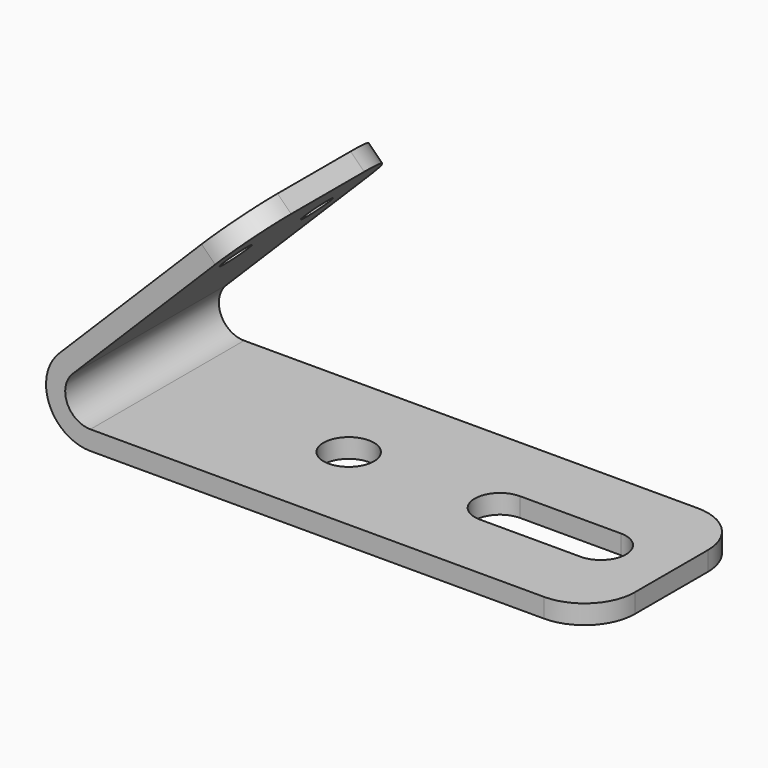
from build123d import *

# Parameters (mm, degrees)
F0_W     = 50
F0_H     = 1.9
F1_DEPTH = 19.05
F3_DEPTH = 1.901
F4_D     = 5
F4_DEPTH = 1.901
F5_R     = 1.5
F6_DEPTH = 15.3122698372
F7_R     = 5


with BuildPart() as f1:
    # F0 (on Front) → F1 (new body)
    with BuildSketch(Plane.XZ):
        with Locations((25, 0.95)):
            Rectangle(F0_W, F0_H)
        with BuildLine():
            ThreePointArc((-3.1112698372, 7.5112698372), (-4.065069943, 2.7161928976), (0, 0))
            Line((0, 0), (0, 1.9))
            ThreePointArc((0, 1.9), (-2.3096988313, 3.4432914191), (-1.767766953, 6.167766953))
            Line((-1.767766953, 6.167766953), (15.9099025767, 23.8454364826))
            Line((15.9099025767, 23.8454364826), (14.5663996924, 25.1889393669))
            Line((14.5663996924, 25.1889393669), (-3.1112698372, 7.5112698372))
        make_face()
    extrude(amount=F1_DEPTH)

    # F2 (on face) → F3 (cut, through all)
    with BuildSketch(Plane.XY.offset(1.9)):
        with BuildLine():
            Line((33, -12.025), (43, -12.025))
            ThreePointArc((43, -12.025), (45.5, -9.525), (43, -7.025))
            Line((43, -7.025), (33, -7.025))
            ThreePointArc((33, -7.025), (30.5, -9.525), (33, -12.025))
        make_face()
    extrude(amount=-F3_DEPTH, mode=Mode.SUBTRACT)

    # F4 (through all, one way)
    with BuildSketch(Plane.XY.offset(1.9)):
        with Locations((18, -9.525)):
            Circle(F4_D / 2)
    extrude(amount=-F4_DEPTH, mode=Mode.SUBTRACT)

    # F5 (on face) → F6 (cut, through all)
    with BuildSketch(Plane(origin=(-3.967766953, 0, 3.967766953), x_dir=(0, 1, 0), z_dir=(0.7071067812, 0, -0.7071067812))):
        with Locations((-14.55, 20.9112698372)):
            Circle(F5_R)
        with Locations((-4.5, 20.9112698372)):
            Circle(F5_R)
    extrude(amount=-F6_DEPTH, mode=Mode.SUBTRACT)

    # F7
    f7_edges = [f1.edges().sort_by_distance(p)[0] for p in [
        (50, 0, 0.95),
        (50, -19.05, 0.95),
        (15.238151, -19.05, 24.517188),
        (15.238151, 0, 24.517188),
    ]]
    fillet(f7_edges, radius=F7_R)


solid = f1.part
